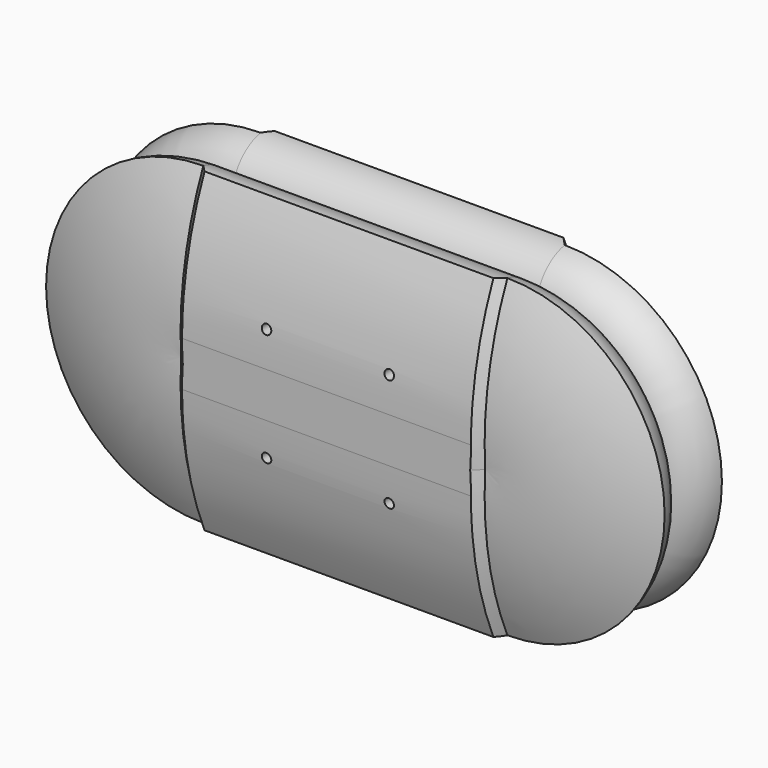
from build123d import *

# Parameters (mm, degrees)
F0_W        = 101.5806943178
F0_H        = 48.01966995
F1_DEPTH    = 105.5511329323
F2_R        = 29.2525430431
F3_T1_DEPTH = 554.2240944956
F4_SIZE     = 5.08
F5_T2_ANGLE = 31.2878347999
F7_D        = 6.35
F9_ANGLE    = 180


# Not quite as in the source:
# - a fillet or chamfer that OpenCascade refuses, or shapes differently, is made with other operations: its cross-section is extruded or revolved along the edge and cut away or added


with BuildPart() as f1:
    # F0 (on Top) → F1 (new body)
    with BuildSketch(Plane.XY):
        with Locations((9.8017528653, 24.009834975)):
            Rectangle(F0_W, F0_H)
    extrude(amount=F1_DEPTH)

    # F2
    f2_edges = [f1.edges().sort_by_distance(p)[0] for p in [
        (9.801753, 0, 105.551133),
    ]]
    fillet(f2_edges, radius=F2_R)

    # F3: fillet of radius 227.7292364389 on 1 edges, made by hand

    # F3_s2 → F3_t1 (cut)
    with BuildSketch(Plane.YZ.offset(-267.3102943825)):
        with BuildLine():
            ThreePointArc((29.2525430431, 105.5511329323), (43.2785349621, 61.2491955933), (48.01966995, 15.0224528968))
            Line((48.01966995, 15.0224528968), (48.01966995, 105.5511329323))
            Line((48.01966995, 105.5511329323), (29.2525430431, 105.5511329323))
        make_face()
    extrude(amount=F3_T1_DEPTH, mode=Mode.SUBTRACT)

    # F4
    f4_edges = [f1.edges().sort_by_distance(p)[0] for p in [
        (9.801753, 0, 0),
    ]]
    chamfer(f4_edges, length=F4_SIZE)

    # F5: chamfer of 5.08 on 1 edges, made by hand

    # F5_s1 → F5_t2 (revolve, cut)
    with BuildSketch(Plane(origin=(0, -44.077363084, 85.1947407747), x_dir=(1, 0, 0), z_dir=(0, -0.4595143579, 0.8881703411))):
        with BuildLine():
            Line((61.6697307588, 68.8619315298), (54.4344692897, 76.0971929988))
            Line((54.4344692897, 76.0971929988), (54.4344692897, 76.8591929988))
            ThreePointArc((54.4344692897, 76.8591929988), (57.513284657, 75.7815622643), (60.5921000242, 75.7815622643))
            Line((60.5921000242, 75.7815622643), (61.3541000242, 75.0195622643))
            ThreePointArc((61.3541000242, 75.0195622643), (61.3541000242, 71.9407468971), (62.4317307588, 68.8619315298))
            Line((62.4317307588, 68.8619315298), (61.6697307588, 68.8619315298))
        make_face()
    revolve(axis=Axis((60.5921000242, -179.7095664878, 15.022452897), (-1, 0, 0)), revolution_arc=F5_T2_ANGLE, mode=Mode.SUBTRACT)

    # F7 (through all)
    with Locations(Plane.XZ):
        with Locations((0, 37.8390811384)):
            Hole(F7_D / 2)

    # F8: F1 across plane


with BuildPart() as f1_1:
    add(f1.part)
    add(f1.part.mirror(Plane.XZ))

    # F8_face (on face) → F9 (revolve)
    with BuildSketch(Plane(origin=(60.5921000242, 0, 46.1455237947), x_dir=(0, 1, 0), z_dir=(1, 0, 0))):
        with BuildLine():
            Line((0, -41.0655237947), (5.08, -46.1455237947))
            Line((5.08, -46.1455237947), (42.432298984, -46.1455237947))
            ThreePointArc((42.432298984, -46.1455237947), (39.5623129602, 7.5101449883), (23.9216912378, 58.9157727391))
            ThreePointArc((23.9216912378, 58.9157727391), (6.7619645003, 48.8582833159), (0, 30.1530660945))
            ThreePointArc((0, 30.1530660945), (-6.7619645003, 48.8582833159), (-23.9216912378, 58.9157727391))
            ThreePointArc((-23.9216912378, 58.9157727391), (-39.5623129602, 7.5101449883), (-42.432298984, -46.1455237947))
            Line((-42.432298984, -46.1455237947), (-5.08, -46.1455237947))
            Line((-5.08, -46.1455237947), (0, -41.0655237947))
        make_face()
    revolve(axis=Axis((60.5921000242, -23.756149492, 0), (0, 1, 0)), revolution_arc=F9_ANGLE)

    # F10: F1 across face


with BuildPart() as f1_2:
    add(f1_1.part)
    add(f1_1.part.mirror(Plane(origin=(9.6264102551, 26.4795740308, 0), x_dir=(1, 0, 0), z_dir=(0, 0, -1))))

    # F11: F1 across face


with BuildPart() as f1_3:
    add(f1_2.part)
    add(f1_2.part.mirror(Plane(origin=(-40.9885942936, 0, 0), x_dir=(0, -1, 0), z_dir=(-1, 0, 0))))


solid = f1_3.part
